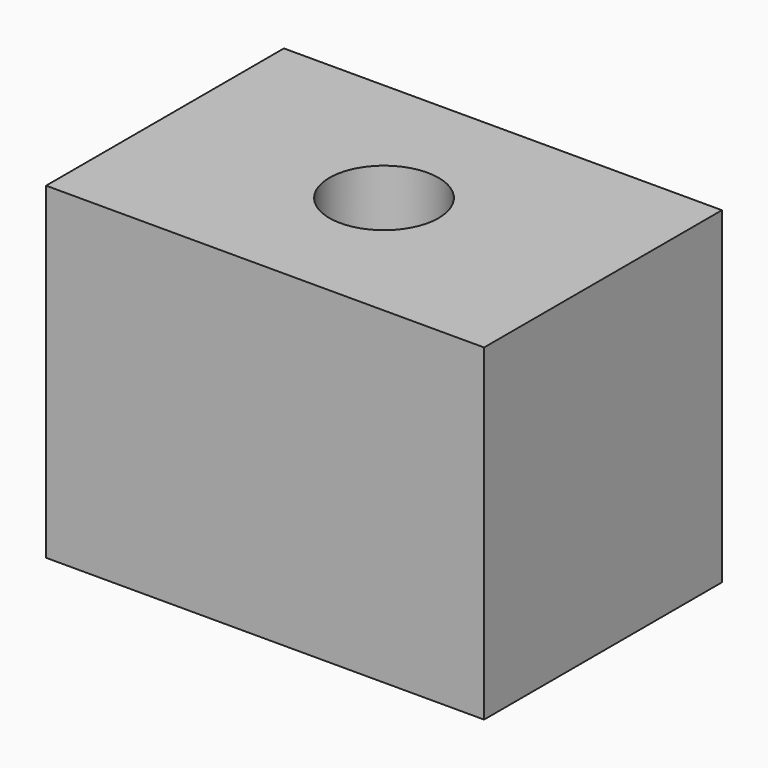
from build123d import *

# Parameters (mm, degrees)
F0_R          = 19.05
F0_R_2        = 7.9375
F1_DEPTH      = 25.4
F3_W          = 16.0429216921
F3_H          = 10.8887040988
F3_R          = 2
F4_DEPTH      = 6
F4_DEPTH_BACK = 6


# Not quite as in the source:
# - the program builds the solid bodies; features that only make, move or delete a surface that nothing else refers to are left out


with BuildPart() as f1:
    # F0 (on Top) → F1 (new body)
    with BuildSketch(Plane.XY):
        Circle(F0_R)
        Circle(F0_R_2, mode=Mode.SUBTRACT)
    extrude(amount=F1_DEPTH)


with BuildPart() as f4:
    # F3 (on Top) → F4 (new body, two sides)
    with BuildSketch(Plane.XY) as f4_sk:
        Rectangle(F3_W, F3_H)
        Circle(F3_R, mode=Mode.SUBTRACT)
    extrude(amount=F4_DEPTH)
    extrude(f4_sk.sketch, amount=-F4_DEPTH_BACK)


solid = f4.part
